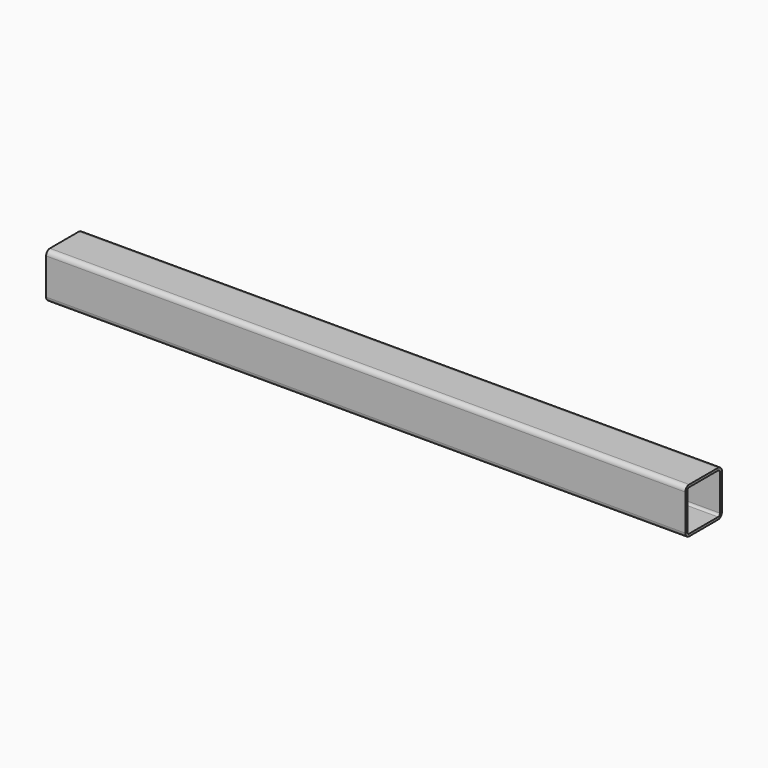
from build123d import *

# Parameters (mm, degrees)
F2_DEPTH = 444.5
F3_ANGLE = 90


# Not quite as in the source:
# - a variable given as a bare number and used for a length is read in inches; the dataset says mm whatever the document's units were


with BuildPart() as f2:
    # F0 (on Top) → F2 (new body)
    with BuildSketch(Plane.XY):
        with BuildLine():
            Line((-12.573, -15.875), (12.573, -15.875))
            ThreePointArc((12.573, -15.875), (14.9078665915, -14.9078665915), (15.875, -12.573))
            Line((15.875, -12.573), (15.875, 12.573))
            ThreePointArc((15.875, 12.573), (14.9078665915, 14.9078665915), (12.573, 15.875))
            Line((12.573, 15.875), (-12.573, 15.875))
            ThreePointArc((-12.573, 15.875), (-14.9078665915, 14.9078665915), (-15.875, 12.573))
            Line((-15.875, 12.573), (-15.875, -12.573))
            ThreePointArc((-15.875, -12.573), (-14.9078665915, -14.9078665915), (-12.573, -15.875))
        make_face()
        with BuildLine():
            Line((-12.573, 14.224), (12.573, 14.224))
            ThreePointArc((12.573, 14.224), (13.7404332957, 13.7404332957), (14.224, 12.573))
            Line((14.224, 12.573), (14.224, -12.573))
            ThreePointArc((14.224, -12.573), (13.7404332957, -13.7404332957), (12.573, -14.224))
            Line((12.573, -14.224), (-12.573, -14.224))
            ThreePointArc((-12.573, -14.224), (-13.7404332957, -13.7404332957), (-14.224, -12.573))
            Line((-14.224, -12.573), (-14.224, 12.573))
            ThreePointArc((-14.224, 12.573), (-13.7404332957, 13.7404332957), (-12.573, 14.224))
        make_face(mode=Mode.SUBTRACT)
    extrude(amount=F2_DEPTH)


with BuildPart() as f2_1:
    # F3: moved
    add(f2.part.rotate(Axis((-15.875, 0, 444.5), (0, 1, 0)), F3_ANGLE))


solid = f2_1.part
